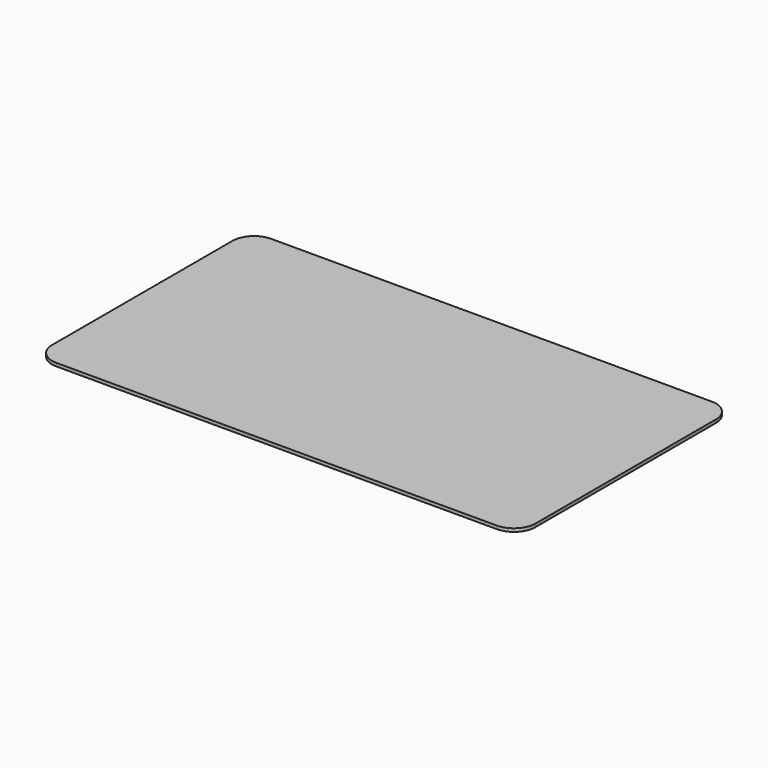
from build123d import *

# Parameters (mm, degrees)
F1_W     = 90
F1_H     = 50
F2_DEPTH = 0.6
F3_R     = 4


with BuildPart() as f2:
    # F1 (on Top) → F2 (new body)
    with BuildSketch(Plane.XY):
        Rectangle(F1_W, F1_H)
    extrude(amount=F2_DEPTH)

    # F3
    f3_edges = [f2.edges().sort_by_distance(p)[0] for p in [
        (-45, 25, 0.3),
        (45, 25, 0.3),
        (45, -25, 0.3),
        (-45, -25, 0.3),
    ]]
    fillet(f3_edges, radius=F3_R)


solid = f2.part
